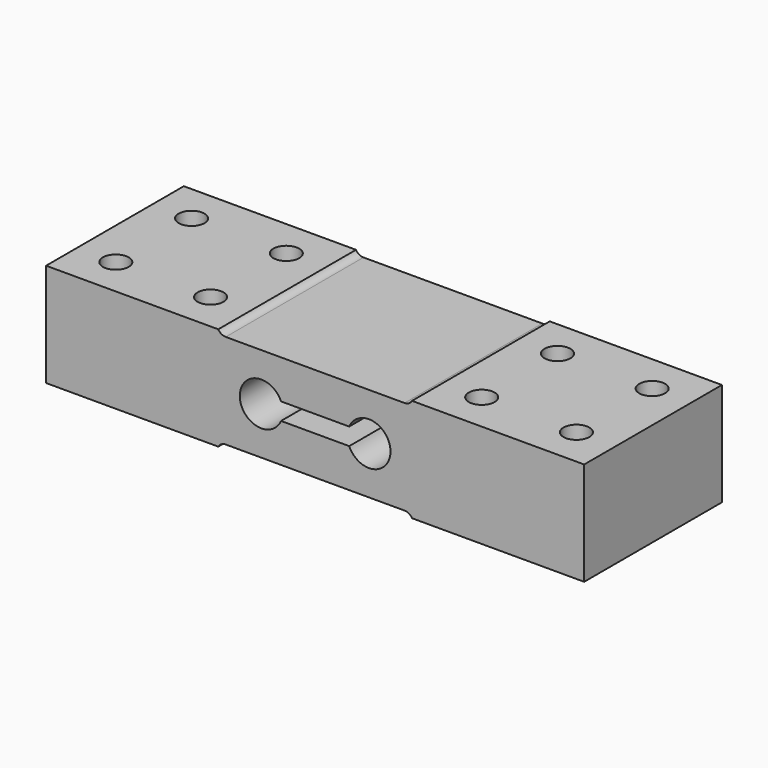
from build123d import *

# Parameters (mm, degrees)
F0_W        = 125
F0_H        = 40
F0_R        = 3
F1_DEPTH    = 24
F3_DEPTH    = 45
F4_W        = 45
F4_H        = 40
F5_DEPTH    = 1
F6_W        = 45
F6_H        = 40
F7_DEPTH    = 1
F8_T1_DEPTH = 40


# Not quite as in the source:
# - a fillet or chamfer that OpenCascade refuses, or shapes differently, is made with other operations: its cross-section is extruded or revolved along the edge and cut away or added


with BuildPart() as f1:
    # F0 (on Top) → F1 (new body)
    with BuildSketch(Plane.XY):
        with Locations((62.5, 20)):
            Rectangle(F0_W, F0_H)
        with Locations((9, 9)):
            Circle(F0_R, mode=Mode.SUBTRACT)
        with Locations((31, 9)):
            Circle(F0_R, mode=Mode.SUBTRACT)
        with Locations((94, 9)):
            Circle(F0_R, mode=Mode.SUBTRACT)
        with Locations((116, 9)):
            Circle(F0_R, mode=Mode.SUBTRACT)
        with Locations((9, 31)):
            Circle(F0_R, mode=Mode.SUBTRACT)
        with Locations((31, 31)):
            Circle(F0_R, mode=Mode.SUBTRACT)
        with Locations((94, 31)):
            Circle(F0_R, mode=Mode.SUBTRACT)
        with Locations((116, 31)):
            Circle(F0_R, mode=Mode.SUBTRACT)
    extrude(amount=F1_DEPTH)

    # F2 (on face) → F3 (cut)
    with BuildSketch(Plane.XZ):
        with BuildLine():
            Line((54, 14), (54.582575695, 14))
            ThreePointArc((54.582575695, 14), (45, 12), (54.582575695, 10))
            Line((54.582575695, 10), (54, 10))
            Line((54, 10), (54, 14))
        make_face()
        with BuildLine():
            ThreePointArc((54.582575695, 10), (54.8945315647, 10.9784517816), (55, 12))
            ThreePointArc((55, 12), (54.8945315647, 13.0215482184), (54.582575695, 14))
            Line((54.582575695, 14), (54, 14))
            Line((54, 14), (54, 10))
            Line((54, 10), (54.582575695, 10))
        make_face()
        with BuildLine():
            ThreePointArc((54.582575695, 14), (54.8945315647, 13.0215482184), (55, 12))
            ThreePointArc((55, 12), (54.8945315647, 10.9784517816), (54.582575695, 10))
            Line((54.582575695, 10), (70.417424305, 10))
            ThreePointArc((70.417424305, 10), (70, 12), (70.417424305, 14))
            Line((70.417424305, 14), (54.582575695, 14))
        make_face()
        with BuildLine():
            Line((71, 14), (70.417424305, 14))
            ThreePointArc((70.417424305, 14), (70, 12), (70.417424305, 10))
            Line((70.417424305, 10), (71, 10))
            Line((71, 10), (71, 14))
        make_face()
        with BuildLine():
            ThreePointArc((80, 12), (76.0215482184, 16.8945315647), (70.417424305, 14))
            Line((70.417424305, 14), (71, 14))
            Line((71, 14), (71, 10))
            Line((71, 10), (70.417424305, 10))
            ThreePointArc((70.417424305, 10), (76.0215482184, 7.1054684353), (80, 12))
        make_face()
    extrude(amount=-F3_DEPTH, mode=Mode.SUBTRACT)

    # F4 (on face) → F5 (cut)
    with BuildSketch(Plane.XY.offset(24)):
        with Locations((62.5, 20)):
            Rectangle(F4_W, F4_H)
    extrude(amount=-F5_DEPTH, mode=Mode.SUBTRACT)

    # F6 (on face) → F7 (cut)
    with BuildSketch(Plane(origin=(0, 0, 0), x_dir=(1, 0, 0), z_dir=(0, 0, -1))):
        with Locations((62.5, -20)):
            Rectangle(F6_W, F6_H)
    extrude(amount=-F7_DEPTH, mode=Mode.SUBTRACT)

    # F8: fillet of radius 2 on 4 edges, made by hand

    # F8_s2 → F8_t1 (join)
    with BuildSketch(Plane.XZ.offset(-40)):
        with BuildLine():
            ThreePointArc((41.7320508076, 1), (40.7320508076, 0.7320508076), (40, 0))
            Line((40, 0), (40, 1))
            Line((40, 1), (41.7320508076, 1))
        make_face()
        with BuildLine():
            ThreePointArc((85, 0), (84.2679491924, 0.7320508076), (83.2679491924, 1))
            Line((83.2679491924, 1), (85, 1))
            Line((85, 1), (85, 0))
        make_face()
        with BuildLine():
            ThreePointArc((83.2679491924, 23), (84.2679491924, 23.2679491924), (85, 24))
            Line((85, 24), (85, 23))
            Line((85, 23), (83.2679491924, 23))
        make_face()
        with BuildLine():
            ThreePointArc((40, 24), (40.7320508076, 23.2679491924), (41.7320508076, 23))
            Line((41.7320508076, 23), (40, 23))
            Line((40, 23), (40, 24))
        make_face()
    extrude(amount=F8_T1_DEPTH)


solid = f1.part
